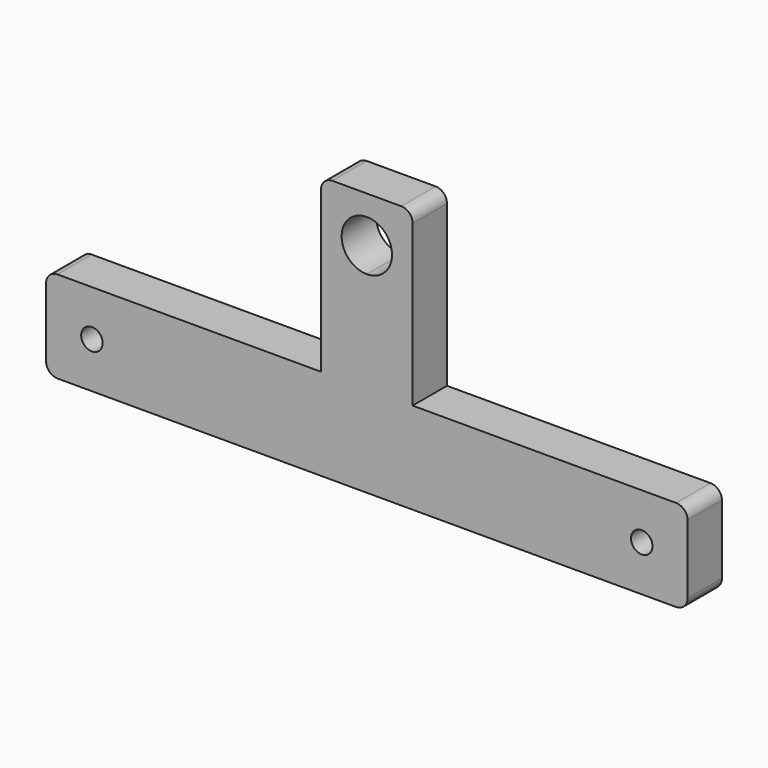
from build123d import *

# Parameters (mm, degrees)
F0_R     = 1.190625
F1_DEPTH = 4.7625
F2_R     = 1.27


# Not quite as in the source:
# - a feature names something its author has since deleted; it is built from what else it names


with BuildPart() as f1:
    # F0 (on Front) → F1 (new body)
    with BuildSketch(Plane.XZ):
        with BuildLine():
            Line((0, 5.08), (5.08, 5.08))
            Line((5.08, 5.08), (5.08, 14.605))
            Line((5.08, 14.605), (5.08, 24.13))
            Line((5.08, 24.13), (0, 24.13))
            Line((0, 24.13), (0, 21.844))
            ThreePointArc((0, 21.844), (1.9756563466, 21.0256563466), (2.794, 19.05))
            ThreePointArc((2.794, 19.05), (1.9756563466, 17.0743436534), (0, 16.256))
            Line((0, 16.256), (0, 5.08))
        make_face()
        with BuildLine():
            Line((-5.08, 5.08), (0, 5.08))
            Line((0, 5.08), (0, 16.256))
            ThreePointArc((0, 16.256), (-2.794, 19.05), (0, 21.844))
            Line((0, 21.844), (0, 24.13))
            Line((0, 24.13), (-5.08, 24.13))
            Line((-5.08, 24.13), (-5.08, 5.08))
        make_face()
        Polygon((35.56, -5.08), (35.56, 5.08), (5.08, 5.08), (0, 5.08), (-5.08, 5.08), (-35.56, 5.08), (-35.56, -5.08), align=None)
        with Locations((-30.48, 0)):
            Circle(F0_R, mode=Mode.SUBTRACT)
        with Locations((30.48, 0)):
            Circle(F0_R, mode=Mode.SUBTRACT)
    extrude(amount=F1_DEPTH)

    # F2
    f2_edges = [f1.edges().sort_by_distance(p)[0] for p in [
        (-5.08, -2.38125, 24.13),
        (5.08, -2.38125, 24.13),
        (35.56, -2.38125, 5.08),
        (35.56, -2.38125, -5.08),
        (-35.56, -2.38125, -5.08),
        (-35.56, -2.38125, 5.08),
    ]]
    fillet(f2_edges, radius=F2_R)


solid = f1.part
